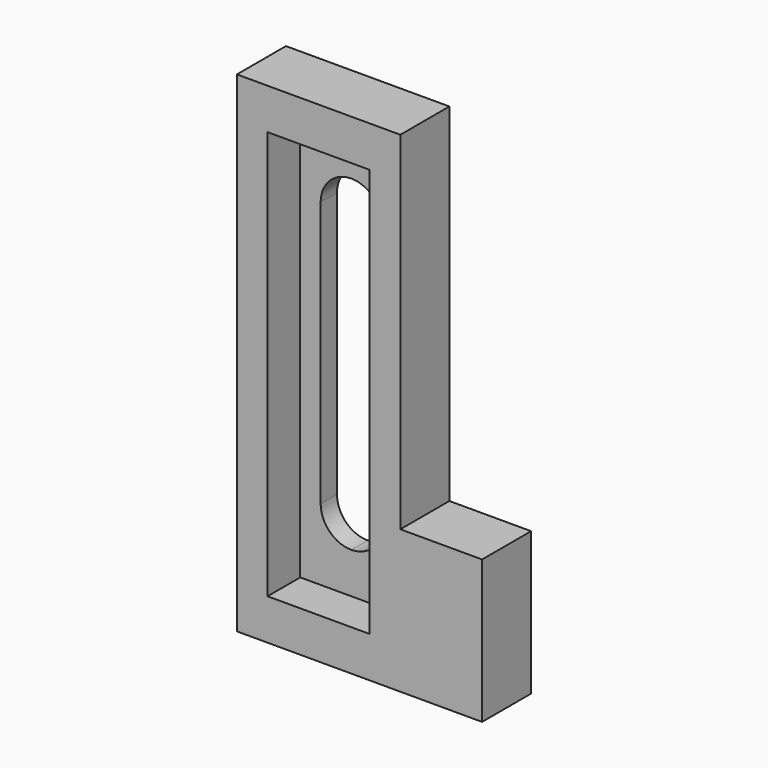
from build123d import *

# Parameters (mm, degrees)
F0_W     = 25
F0_H     = 100
F0_W_2   = 15
F0_H_2   = 80
F1_DEPTH = 15
F2_DEPTH = 10
F3_DEPTH = 15.001
F4_R     = 7.49999


# Not quite as in the source:
# - a fillet or chamfer is up to 0.001 mm smaller than in the source, because OpenCascade refuses the exact size


with BuildPart() as f1:
    # F0 (on Front) → F1 (new body)
    with BuildSketch(Plane.XZ):
        Polygon((20, -25), (20, 60), (-20, 60), (-20, -60), (40, -60), (40, -25), align=None)
        Rectangle(F0_W, F0_H, mode=Mode.SUBTRACT)
        Rectangle(F0_W, F0_H)
        Rectangle(F0_W_2, F0_H_2, mode=Mode.SUBTRACT)
        Rectangle(F0_W_2, F0_H_2)
    extrude(amount=-F1_DEPTH)

    # F0 (on Front) → F2 (cut)
    with BuildSketch(Plane.XZ):
        Rectangle(F0_W, F0_H)
        Rectangle(F0_W_2, F0_H_2, mode=Mode.SUBTRACT)
    extrude(amount=-F2_DEPTH, mode=Mode.SUBTRACT)

    # F0 (on Front) → F3 (cut, through all)
    with BuildSketch(Plane.XZ):
        Rectangle(F0_W_2, F0_H_2)
    extrude(amount=-F3_DEPTH, mode=Mode.SUBTRACT)

    # F4 (radius 7.5 in the source; OpenCascade refuses exactly that, so slightly less here)
    f4_edges = [f1.edges().sort_by_distance(p)[0] for p in [
        (-7.5, 12.5, 40),
        (7.5, 12.5, 40),
        (-7.5, 12.5, -40),
        (7.5, 12.5, -40),
    ]]
    fillet(f4_edges, radius=F4_R)


solid = f1.part
